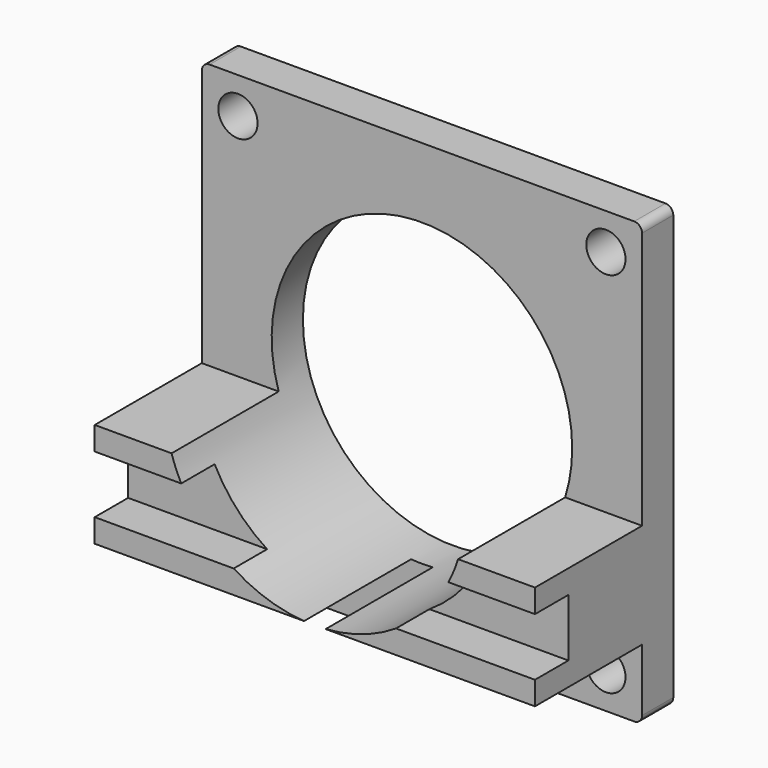
from build123d import *

# Parameters (mm, degrees)
F0_R          = 2.5144921482
F0_R_2        = 19.25
F1_DEPTH      = 5
F4_END_RADIUS = 19.25
F4_REACH      = 78.1652482066


with BuildPart() as f1:
    # F0 (on Front) → F1 (new body)
    with BuildSketch(Plane.XZ):
        with BuildLine():
            Line((-27.2, -28.2), (27.2, -28.2))
            ThreePointArc((27.2, -28.2), (27.9071067812, -27.9071067812), (28.2, -27.2))
            Line((28.2, -27.2), (28.2, 27.2))
            ThreePointArc((28.2, 27.2), (27.9071067812, 27.9071067812), (27.2, 28.2))
            Line((27.2, 28.2), (-27.2, 28.2))
            ThreePointArc((-27.2, 28.2), (-27.9071067812, 27.9071067812), (-28.2, 27.2))
            Line((-28.2, 27.2), (-28.2, -27.2))
            ThreePointArc((-28.2, -27.2), (-27.9071067812, -27.9071067812), (-27.2, -28.2))
        make_face()
        with Locations((-23.57, -23.57)):
            Circle(F0_R, mode=Mode.SUBTRACT)
        with Locations((23.57, -23.57)):
            Circle(F0_R, mode=Mode.SUBTRACT)
        with Locations((-23.57, 23.57)):
            Circle(F0_R, mode=Mode.SUBTRACT)
        Circle(F0_R_2, mode=Mode.SUBTRACT)
        with Locations((23.57, 23.57)):
            Circle(F0_R, mode=Mode.SUBTRACT)
    extrude(amount=F1_DEPTH)

    f4_end = (Plane.ZX.offset(-2.5) * Cylinder(F4_END_RADIUS, 316.1669127895, mode=Mode.PRIVATE)).faces().sort_by_distance((-19.25, -2.5, 0))[0]
    # F3 (on face) → F4 (join, up to the whole of a round face its end follows)
    with BuildSketch(Plane(origin=(-28.2, 0, 0), x_dir=(0, -1, 0), z_dir=(-1, 0, 0))):
        Polygon((4.9999998882, -16.2), (4.9999998882, -19.2), (22.1499998882, -19.2), (22.1499998882, -16.2), (21.9999998882, -16.2), (16.7999998882, -16.2), (16.7999998882, -8.8), (22.1499998882, -8.8), (22.1499998882, -5.8), (4.9999998882, -5.8), align=None)
    f4_long = extrude(amount=-F4_REACH, mode=Mode.PRIVATE)
    add(split(f4_long, bisect_by=f4_end, keep=Keep.ALL, mode=Mode.PRIVATE).solids().sort_by_distance((-28.2, -12.347048043, -12.5))[0])

    # F5: F1 across plane


with BuildPart() as f1_1:
    add(f1.part)
    add(f1.part.mirror(Plane.YZ))


solid = f1_1.part
